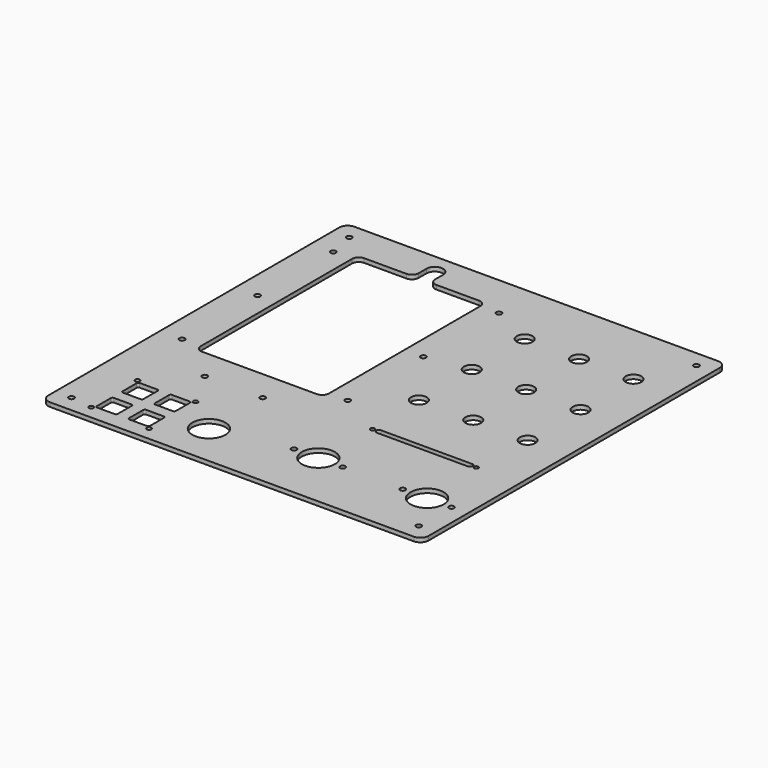
from build123d import *

# Parameters (mm, degrees)
F0_W     = 292.1
F0_H     = 292.1
F0_R     = 2.06375
F1_DEPTH = 3.175
F2_R     = 1.778
F2_W     = 16.0782
F2_H     = 16.0782
F2_R_2   = 2.06375
F2_R_3   = 12.7
F2_R_4   = 6.0325
F2_R_5   = 2.032
F2_R_6   = 1.651
F2_W_2   = 73.787
F2_H_2   = 4.064
F3_DEPTH = 3.176
F4_R     = 5.08
F5_R     = 1.27
F6_R     = 6.35
F7_R     = 1.778


with BuildPart() as f1:
    # F0 (on Top) → F1 (new body)
    with BuildSketch(Plane.XY):
        Rectangle(F0_W, F0_H)
        with Locations((-133.35, -133.35)):
            Circle(F0_R, mode=Mode.SUBTRACT)
        with Locations((133.35, -133.35)):
            Circle(F0_R, mode=Mode.SUBTRACT)
        with Locations((-133.35, 133.35)):
            Circle(F0_R, mode=Mode.SUBTRACT)
        with Locations((133.35, 133.35)):
            Circle(F0_R, mode=Mode.SUBTRACT)
    extrude(amount=-F1_DEPTH)

    # F2 (on face) → F3 (cut, through all)
    with BuildSketch(Plane.XY):
        with BuildLine():
            Line((-114.6175, -37.7825), (-16.1925, -37.7825))
            Line((-16.1925, -37.7825), (-16.1925, 117.7925))
            Line((-16.1925, 117.7925), (-59.055, 117.7925))
            Line((-59.055, 117.7925), (-59.055, 130.4925))
            ThreePointArc((-59.055, 130.4925), (-65.405, 136.8425), (-71.755, 130.4925))
            Line((-71.755, 130.4925), (-71.755, 117.7925))
            Line((-71.755, 117.7925), (-114.6175, 117.7925))
            Line((-114.6175, 117.7925), (-114.6175, -37.7825))
        make_face()
        with Locations((-116.3955, -91.1225)):
            Circle(F2_R)
        with Locations((-71.9455, -91.1225)):
            Circle(F2_R)
        with Locations((-71.9455, -135.5725)):
            Circle(F2_R)
        with Locations((-116.3955, -135.5725)):
            Circle(F2_R)
        with Locations((-106.5784, -100.9396)):
            Rectangle(F2_W, F2_H)
        with Locations((-81.7626, -100.9396)):
            Rectangle(F2_W, F2_H)
        with Locations((-106.5784, -125.7554)):
            Rectangle(F2_W, F2_H)
        with Locations((-81.7626, -125.7554)):
            Rectangle(F2_W, F2_H)
        with Locations((-129.06375, -32.5755)):
            Circle(F2_R_2)
        with Locations((-1.74625, -32.5755)):
            Circle(F2_R_2)
        with Locations((31.242, -102.108)):
            Circle(F2_R_3)
        with Locations((114.808, -102.108)):
            Circle(F2_R_3)
        with Locations((31.242, 96.012)):
            Circle(F2_R_4)
        with Locations((31.242, 45.212)):
            Circle(F2_R_4)
        with Locations((31.242, -5.588)):
            Circle(F2_R_4)
        with Locations((73.025, 96.012)):
            Circle(F2_R_4)
        with Locations((73.025, 45.212)):
            Circle(F2_R_4)
        with Locations((73.025, -5.588)):
            Circle(F2_R_4)
        with Locations((114.808, 96.012)):
            Circle(F2_R_4)
        with Locations((114.808, 45.212)):
            Circle(F2_R_4)
        with Locations((114.808, -5.588)):
            Circle(F2_R_4)
        with Locations((-43.815, -113.3475)):
            Circle(F2_R_3)
        with Locations((12.51585, -102.108)):
            Circle(F2_R_5)
        with Locations((49.96815, -102.108)):
            Circle(F2_R_5)
        with Locations((96.08185, -102.108)):
            Circle(F2_R_5)
        with Locations((133.53415, -102.108)):
            Circle(F2_R_5)
        with Locations((-129.06375, 112.5855)):
            Circle(F2_R_2)
        with Locations((-1.74625, 112.5855)):
            Circle(F2_R_2)
        with Locations((-129.06375, 40.005)):
            Circle(F2_R_2)
        with Locations((-1.74625, 40.005)):
            Circle(F2_R_2)
        with Locations((33.20415, -52.4891)):
            Circle(F2_R_6)
        with Locations((112.84585, -52.4891)):
            Circle(F2_R_6)
        with Locations((-88.265, -61.75375)):
            Circle(F2_R_2)
        with Locations((-43.815, -61.75375)):
            Circle(F2_R_2)
        with Locations((73.025, -52.4891)):
            Rectangle(F2_W_2, F2_H_2)
    extrude(amount=-F3_DEPTH, mode=Mode.SUBTRACT)

    # F4
    f4_edges = [f1.edges().sort_by_distance(p)[0] for p in [
        (-114.6175, 117.7925, -1.5875),
        (-16.1925, 117.7925, -1.5875),
        (-16.1925, -37.7825, -1.5875),
        (-114.6175, -37.7825, -1.5875),
        (-59.055, 117.7925, -1.5875),
        (-71.755, 117.7925, -1.5875),
    ]]
    fillet(f4_edges, radius=F4_R)

    # F5
    f5_edges = [f1.edges().sort_by_distance(p)[0] for p in [
        (-114.6175, -92.9005, -1.5875),
        (-89.8017, -92.9005, -1.5875),
        (-89.8017, -117.7163, -1.5875),
        (-114.6175, -117.7163, -1.5875),
        (-98.5393, -92.9005, -1.5875),
        (-73.7235, -92.9005, -1.5875),
        (-98.5393, -117.7163, -1.5875),
        (-73.7235, -117.7163, -1.5875),
        (-73.7235, -133.7945, -1.5875),
        (-73.7235, -108.9787, -1.5875),
        (-98.5393, -108.9787, -1.5875),
        (-98.5393, -133.7945, -1.5875),
        (-114.6175, -133.7945, -1.5875),
        (-114.6175, -108.9787, -1.5875),
        (-89.8017, -108.9787, -1.5875),
        (-89.8017, -133.7945, -1.5875),
    ]]
    fillet(f5_edges, radius=F5_R)

    # F6
    f6_edges = [f1.edges().sort_by_distance(p)[0] for p in [
        (-146.05, 146.05, -1.5875),
        (146.05, 146.05, -1.5875),
        (146.05, -146.05, -1.5875),
        (-146.05, -146.05, -1.5875),
    ]]
    fillet(f6_edges, radius=F6_R)

    # F7
    f7_edges = [f1.edges().sort_by_distance(p)[0] for p in [
        (36.1315, -50.4571, -1.5875),
        (109.9185, -50.4571, -1.5875),
        (109.9185, -54.5211, -1.5875),
        (36.1315, -54.5211, -1.5875),
    ]]
    fillet(f7_edges, radius=F7_R)


solid = f1.part
